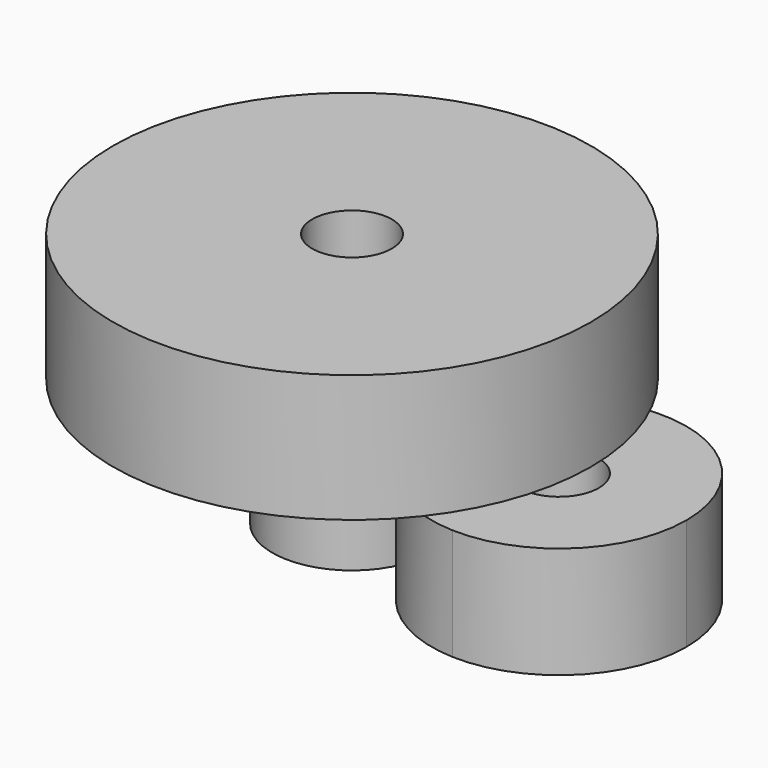
from build123d import *

# Parameters (mm, degrees)
F0_R     = 5
F0_R_2   = 2.5
F1_DEPTH = 8
F2_R     = 15
F2_R_2   = 5
F2_R_3   = 2.5
F3_DEPTH = 8
F4_DEPTH = 7


# Not quite as in the source:
# - a feature names something its author has since deleted; it is built from what else it names


with BuildPart() as f1:
    # F0 (on Top) → F1 (new body)
    with BuildSketch(Plane.XY):
        with Locations((-21, -35.0552037954)):
            Circle(F0_R)
        with Locations((-21, -35.0552037954)):
            Circle(F0_R_2, mode=Mode.SUBTRACT)
    extrude(amount=F1_DEPTH)

    # F2 (on face) → F3 (join)
    with BuildSketch(Plane.XY.offset(8)):
        with Locations((-21, -35.0552037954)):
            Circle(F2_R)
        with Locations((-21, -35.0552037954)):
            Circle(F2_R_2, mode=Mode.SUBTRACT)
        with Locations((-21, -35.0552037954)):
            Circle(F2_R_2)
        with Locations((-21, -35.0552037954)):
            Circle(F2_R_3, mode=Mode.SUBTRACT)
    extrude(amount=F3_DEPTH)

    # F0 (on Top) → F4 (join)
    with BuildSketch(Plane.XY):
        with BuildLine():
            ThreePointArc((-6.0865384615, -36.6641366532), (-10.5, -35.0552037954), (-6.0865384615, -33.4462709377))
            ThreePointArc((-6.0865384615, -33.4462709377), (-6.832708382, -30.1269334892), (-8.3076923077, -27.0611231451))
            ThreePointArc((-8.3076923077, -27.0611231451), (-13.764613537, -29.5082018332), (-16, -35.0552037954))
            ThreePointArc((-16, -35.0552037954), (-13.764613537, -40.6022057577), (-8.3076923077, -43.0492844458))
            ThreePointArc((-8.3076923077, -43.0492844458), (-6.832708382, -39.9834741017), (-6.0865384615, -36.6641366532))
        make_face()
        with BuildLine():
            ThreePointArc((-8.3076923077, -27.0611231451), (-6.832708382, -30.1269334892), (-6.0865384615, -33.4462709377))
            ThreePointArc((-6.0865384615, -33.4462709377), (-5.6512073478, -34.1989485316), (-5.5, -35.0552037954))
            ThreePointArc((-5.5, -35.0552037954), (-5.6512073478, -35.9114590593), (-6.0865384615, -36.6641366532))
            ThreePointArc((-6.0865384615, -36.6641366532), (-6.832708382, -39.9834741017), (-8.3076923077, -43.0492844458))
            ThreePointArc((-8.3076923077, -43.0492844458), (-2.4529980377, -40.8198173324), (0, -35.0552037954))
            ThreePointArc((0, -35.0552037954), (-2.4529980377, -29.2905902584), (-8.3076923077, -27.0611231451))
        make_face()
    extrude(amount=F4_DEPTH)


solid = f1.part
